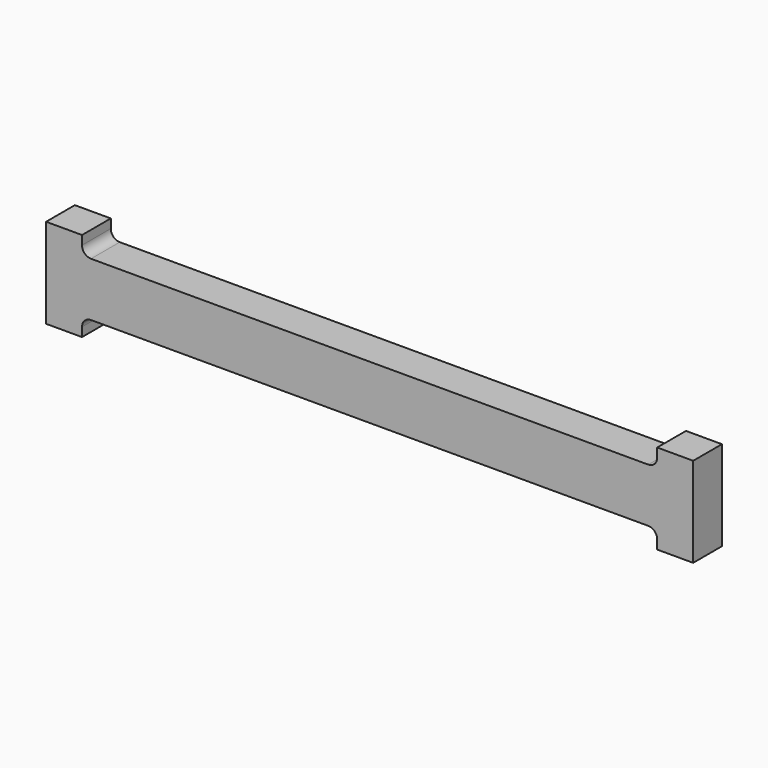
from build123d import *

# Parameters (mm, degrees)
F1_DEPTH = 1
F4_DEPTH = 30
F5_DEPTH = 30


with BuildPart() as f1:
    # F0 (on Front) → F1 (new body, symmetric)
    with BuildSketch(Plane.XZ):
        with BuildLine():
            Line((-16, 2.5), (-18, 2.5))
            Line((-18, 2.5), (-18, 0))
            Line((-18, 0), (0, 0))
            Line((0, 0), (0, 1.5))
            Line((0, 1.5), (-15.5, 1.5))
            ThreePointArc((-15.5, 1.5), (-15.8535533906, 1.6464466094), (-16, 2))
            Line((-16, 2), (-16, 2.5))
        make_face()
        with BuildLine():
            Line((0, 1.5), (0, 0))
            Line((0, 0), (18, 0))
            Line((18, 0), (18, 2.5))
            Line((18, 2.5), (16, 2.5))
            Line((16, 2.5), (16, 2))
            ThreePointArc((16, 2), (15.8535533906, 1.6464466094), (15.5, 1.5))
            Line((15.5, 1.5), (0, 1.5))
        make_face()
        with BuildLine():
            Line((0, 0), (-18, 0))
            Line((-18, 0), (-18, -2.5))
            Line((-18, -2.5), (-16, -2.5))
            Line((-16, -2.5), (-16, -2))
            ThreePointArc((-16, -2), (-15.8535533906, -1.6464466094), (-15.5, -1.5))
            Line((-15.5, -1.5), (0, -1.5))
            Line((0, -1.5), (15.5, -1.5))
            ThreePointArc((15.5, -1.5), (15.8535533906, -1.6464466094), (16, -2))
            Line((16, -2), (16, -2.5))
            Line((16, -2.5), (18, -2.5))
            Line((18, -2.5), (18, 0))
            Line((18, 0), (0, 0))
        make_face()
    extrude(amount=F1_DEPTH, both=True)

    # F3 (on offset) → F5 (cut)
    with BuildSketch(Plane.YZ.offset(15)):
        Polygon((0.925000053, -0.25), (0.925000053, 0.25), (0.674999947, 0.25), (0.674999947, 0), (0.674999947, -0.25), align=None)
        Polygon((-0.6768444622, -0.25), (-0.6768444622, 0), (-0.6768444622, 0.25), (-0.9268444622, 0.25), (-0.9268444622, -0.25), align=None)
    extrude(amount=-F5_DEPTH, mode=Mode.SUBTRACT)


with BuildPart() as f4:
    # F3 (on offset) → F4 (new body)
    with BuildSketch(Plane.YZ.offset(15)):
        Polygon((-0.6768444622, -0.25), (-0.6768444622, 0), (-0.6768444622, 0.25), (-0.9268444622, 0.25), (-0.9268444622, -0.25), align=None)
    extrude(amount=-F4_DEPTH)


with BuildPart() as f4b:
    # F3 (on offset) → F4, piece 2 (new body)
    with BuildSketch(Plane.YZ.offset(15)):
        Polygon((0.925000053, -0.25), (0.925000053, 0.25), (0.674999947, 0.25), (0.674999947, 0), (0.674999947, -0.25), align=None)
    extrude(amount=-F4_DEPTH)


solid = Compound([f1.part, f4.part, f4b.part])
